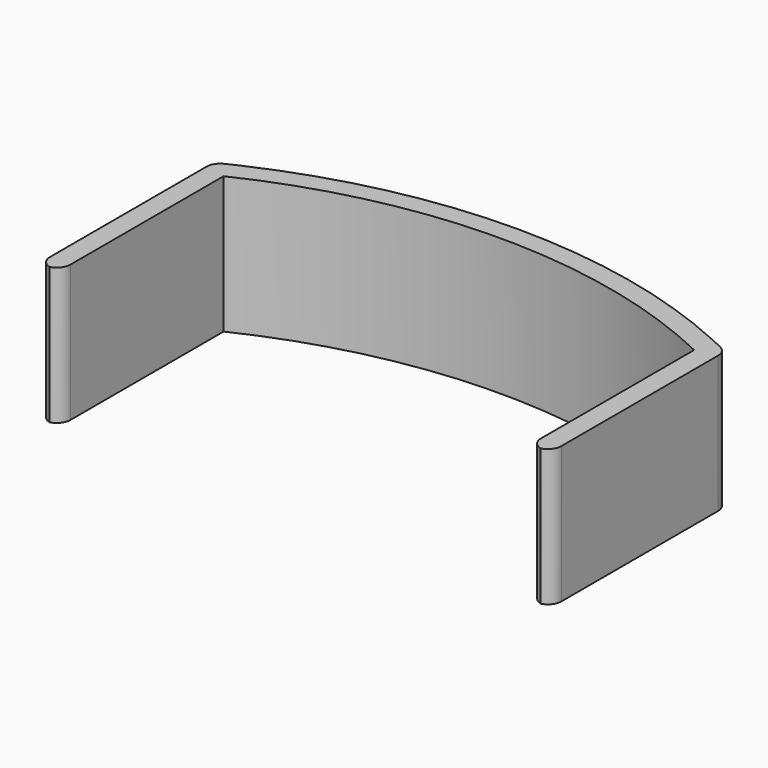
from build123d import *

# Parameters (mm, degrees)
F1_DEPTH    = 12.7
F3_DEPTH    = 32.1945
F4_T1_DEPTH = 19.05
F5_R        = 1.27


# Not quite as in the source:
# - a fillet or chamfer that OpenCascade refuses, or shapes differently, is made with other operations: its cross-section is extruded or revolved along the edge and cut away or added


with BuildPart() as f1:
    # F0 (on Top) → F1 (new body)
    with BuildSketch(Plane.XY):
        with BuildLine():
            Line((-25.9680064888, 45.8637074821), (-25.9680064888, 43.6612258073))
            ThreePointArc((-25.9680064888, 43.6612258073), (-23.9313543809, 44.8099350312), (-21.844, 45.8637074821))
            Line((-21.844, 45.8637074821), (-21.844, 47.9651612006))
            ThreePointArc((-21.844, 47.9651612006), (-23.929083101, 46.9597275008), (-25.9680064888, 45.8637074821))
        make_face()
        with BuildLine():
            ThreePointArc((-21.844, 45.8637074821), (-23.9313543809, 44.8099350312), (-25.9680064888, 43.6612258073))
            Line((-25.9680064888, 43.6612258073), (-25.9680064888, 26.8137074821))
            Line((-25.9680064888, 26.8137074821), (-21.844, 26.8137074821))
            Line((-21.844, 26.8137074821), (-21.844, 45.8637074821))
        make_face()
        with BuildLine():
            ThreePointArc((21.844, 45.8637074821), (23.9313543809, 44.8099350312), (25.9680064888, 43.6612258073))
            Line((25.9680064888, 43.6612258073), (25.9680064888, 45.8637074821))
            ThreePointArc((25.9680064888, 45.8637074821), (23.929083101, 46.9597275008), (21.844, 47.9651612006))
            Line((21.844, 47.9651612006), (21.844, 45.8637074821))
        make_face()
        with BuildLine():
            Line((25.9680064888, 26.8137074821), (25.9680064888, 43.6612258073))
            ThreePointArc((25.9680064888, 43.6612258073), (23.9313543809, 44.8099350312), (21.844, 45.8637074821))
            Line((21.844, 45.8637074821), (21.844, 26.8137074821))
            Line((21.844, 26.8137074821), (25.9680064888, 26.8137074821))
        make_face()
        with BuildLine():
            ThreePointArc((-21.844, 45.8637074821), (0, 50.8), (21.844, 45.8637074821))
            Line((21.844, 45.8637074821), (21.844, 47.9651612006))
            ThreePointArc((21.844, 47.9651612006), (0, 52.705), (-21.844, 47.9651612006))
            Line((-21.844, 47.9651612006), (-21.844, 45.8637074821))
        make_face()
    extrude(amount=F1_DEPTH)

    # F2 (on face) → F3 (cut, symmetric)
    with BuildSketch(Plane.XY.offset(12.7)):
        with BuildLine():
            Line((-23.749, 47.0510576289), (-23.749, 52.2757731378))
            Line((-23.749, 52.2757731378), (-31.0743017153, 52.1406124749))
            Line((-31.0743017153, 52.1406124749), (-30.5507772572, 23.7671602517))
            Line((-30.5507772572, 23.7671602517), (-23.749, 23.7671602517))
            Line((-23.749, 23.7671602517), (-23.749, 26.8137074821))
            Line((-23.749, 26.8137074821), (-25.9680064888, 26.8137074821))
            Line((-25.9680064888, 26.8137074821), (-25.9680064888, 45.8637074821))
            ThreePointArc((-25.9680064888, 45.8637074821), (-24.8655913592, 46.4706293411), (-23.749, 47.0510576289))
        make_face()
        with BuildLine():
            Line((23.749, 52.2757731378), (23.749, 47.0510576289))
            ThreePointArc((23.749, 47.0510576289), (24.8655913592, 46.4706293411), (25.9680064888, 45.8637074821))
            Line((25.9680064888, 45.8637074821), (25.9680064888, 26.8137074821))
            Line((25.9680064888, 26.8137074821), (23.749, 26.8137074821))
            Line((23.749, 26.8137074821), (23.749, 23.7671602517))
            Line((23.749, 23.7671602517), (30.5507772572, 23.7671602517))
            Line((30.5507772572, 23.7671602517), (31.0743017153, 52.1406124749))
            Line((31.0743017153, 52.1406124749), (23.749, 52.2757731378))
        make_face()
        with BuildLine():
            Line((-23.749, 26.8137074821), (-23.749, 47.0510576289))
            ThreePointArc((-23.749, 47.0510576289), (-24.8655913592, 46.4706293411), (-25.9680064888, 45.8637074821))
            Line((-25.9680064888, 45.8637074821), (-25.9680064888, 26.8137074821))
            Line((-25.9680064888, 26.8137074821), (-23.749, 26.8137074821))
        make_face()
        with BuildLine():
            ThreePointArc((25.9680064888, 45.8637074821), (24.8655913592, 46.4706293411), (23.749, 47.0510576289))
            Line((23.749, 47.0510576289), (23.749, 26.8137074821))
            Line((23.749, 26.8137074821), (25.9680064888, 26.8137074821))
            Line((25.9680064888, 26.8137074821), (25.9680064888, 45.8637074821))
        make_face()
    extrude(amount=F3_DEPTH, both=True, mode=Mode.SUBTRACT)

    # F4: fillet of radius 1.27 on 4 edges, made by hand

    # F4_s2 → F4_t1 (cut)
    with BuildSketch(Plane.XY.offset(-3.175)):
        with BuildLine():
            ThreePointArc((-21.844, 28.0837074821), (-22.2159743879, 27.18568187), (-23.114, 26.8137074821))
            Line((-23.114, 26.8137074821), (-21.844, 26.8137074821))
            Line((-21.844, 26.8137074821), (-21.844, 28.0837074821))
        make_face()
        with BuildLine():
            ThreePointArc((-23.749, 28.0837074821), (-23.3770256121, 27.18568187), (-22.479, 26.8137074821))
            Line((-22.479, 26.8137074821), (-23.749, 26.8137074821))
            Line((-23.749, 26.8137074821), (-23.749, 28.0837074821))
        make_face()
        with BuildLine():
            ThreePointArc((23.114, 26.8137074821), (22.2159743879, 27.18568187), (21.844, 28.0837074821))
            Line((21.844, 28.0837074821), (21.844, 26.8137074821))
            Line((21.844, 26.8137074821), (23.114, 26.8137074821))
        make_face()
        with BuildLine():
            ThreePointArc((23.749, 28.0837074821), (23.3770256121, 27.18568187), (22.479, 26.8137074821))
            Line((22.479, 26.8137074821), (23.749, 26.8137074821))
            Line((23.749, 26.8137074821), (23.749, 28.0837074821))
        make_face()
    extrude(amount=F4_T1_DEPTH, mode=Mode.SUBTRACT)

    # F5
    f5_edges = [f1.edges().sort_by_distance(p)[0] for p in [
        (23.749, 47.051058, 6.35),
        (-23.749, 47.051058, 6.35),
    ]]
    fillet(f5_edges, radius=F5_R)


solid = f1.part
